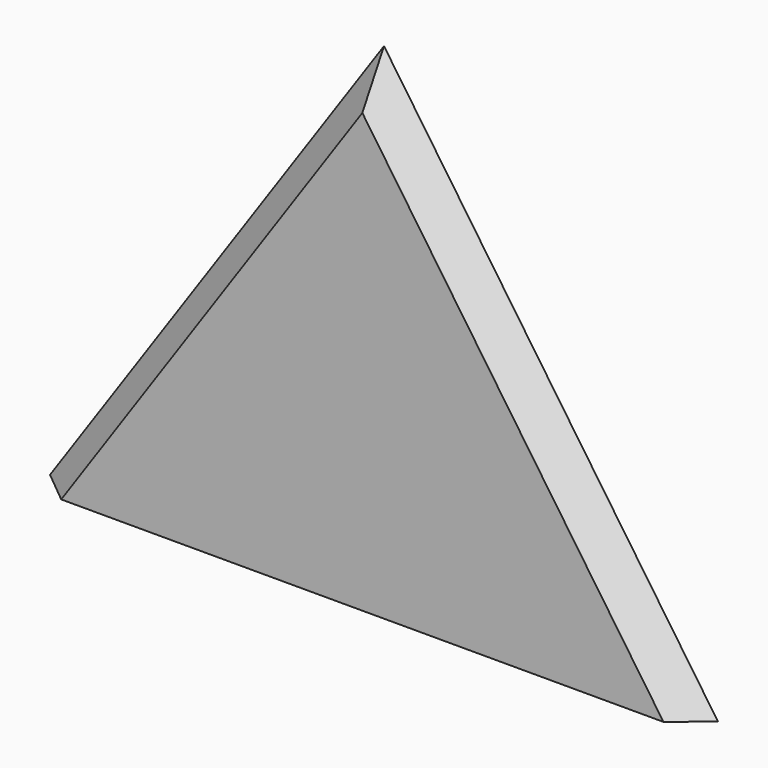
from build123d import *

# Parameters (mm, degrees)
F1_DEPTH    = 1.5
F2_T1_DEPTH = 95.3458705502
F2_T3_DEPTH = 95.3458705502


# Not quite as in the source:
# - a fillet or chamfer that OpenCascade refuses, or shapes differently, is made with other operations: its cross-section is extruded or revolved along the edge and cut away or added


with BuildPart() as f1:
    # F0 (on Front) → F1 (new body, symmetric)
    with BuildSketch(Plane.XZ):
        Polygon((0, 57.386520531), (-39.4333686875, 0), (39.4333686875, 0), align=None)
    extrude(amount=F1_DEPTH, both=True)

    # F2: chamfer of 5 on 2 edges, made by hand

    # F2_s2 → F2_t1 (cut)
    with BuildSketch(Plane(origin=(34.0678617926, 0, 49.578215488), x_dir=(0, 1, 0), z_dir=(-0.5663350853, 0, -0.8241750853))):
        Polygon((3.5, -32.5), (-1.5, -27.5), (-1.5, -32.5), align=None)
    extrude(amount=F2_T1_DEPTH, mode=Mode.SUBTRACT)

    # F2_s4 → F2_t3 (cut)
    with BuildSketch(Plane(origin=(19.9298499385, 0, -29.0034755016), x_dir=(0, 1, 0), z_dir=(-0.5663350853, 0, 0.8241750853))):
        Polygon((3.5, -32.5), (-1.5, -27.5), (-1.5, -32.5), align=None)
    extrude(amount=F2_T3_DEPTH, mode=Mode.SUBTRACT)


solid = f1.part
